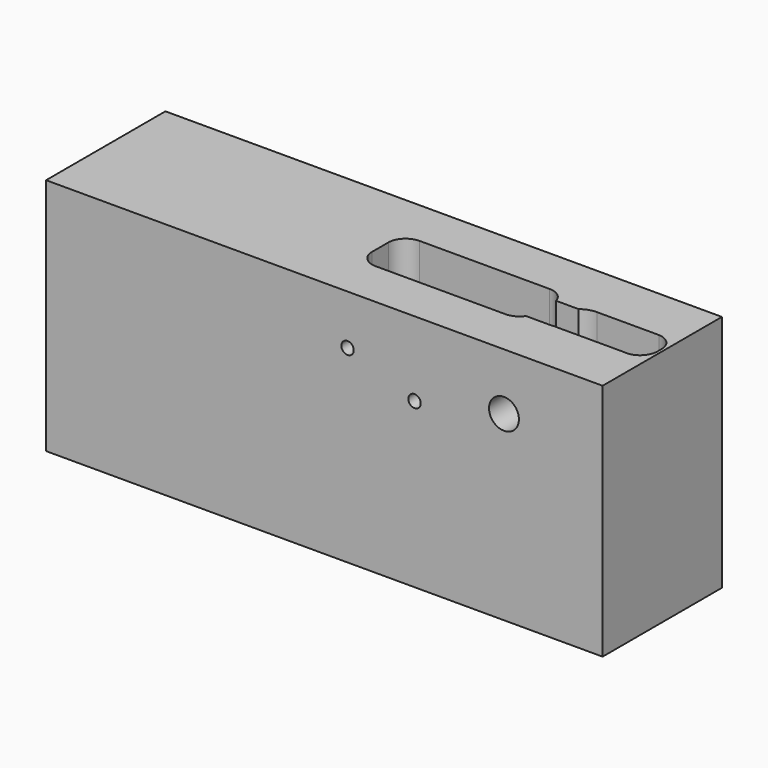
from build123d import *

# Parameters (mm, degrees)
F0_W      = 177.8
F0_H      = 47.6504
F1_DEPTH  = 76.2
F2_R      = 4.7752
F2_R_2    = 1.9812
F3_DEPTH  = 44.45
F5_DEPTH  = 16.002
F7_DEPTH  = 33.528
F9_DEPTH  = 31.7246
F11_DEPTH = 31.7246


# Not quite as in the source:
# - a feature names something its author has since deleted; it is built from what else it names


with BuildPart() as f1:
    # F0 (on Top) → F1 (new body)
    with BuildSketch(Plane.XY):
        with Locations((84.1375, 19.0627)):
            Rectangle(F0_W, F0_H)
    extrude(amount=-F1_DEPTH)

    # F2 (on face) → F3 (cut)
    with BuildSketch(Plane.XZ.offset(4.7625)):
        with Locations((141.5288, -18.1356)):
            Circle(F2_R)
        with Locations((112.9538, -23.8506)):
            Circle(F2_R_2)
        with Locations((91.5416, -15.875)):
            Circle(F2_R_2)
    extrude(amount=-F3_DEPTH, mode=Mode.SUBTRACT)

    # F4 (on face) → F5 (cut)
    with BuildSketch(Plane.XY):
        with BuildLine():
            Line((172.1358, 18.2664336953), (172.1358, 19.8998040895))
            ThreePointArc((172.1358, 19.8998040895), (170.6147547927, 23.7117700549), (166.887268424, 25.4294744577))
            Line((166.887268424, 25.4294744577), (147.1168, 25.4294744577))
            ThreePointArc((147.1168, 25.4294744577), (141.7286463274, 23.1976281303), (139.4968, 17.8094744577))
            Line((139.4968, 17.8094744577), (139.4968, 17.5517135975))
            ThreePointArc((139.4968, 17.5517135975), (140.8917039546, 14.1841175521), (144.2593, 12.7892135975))
            Line((144.2593, 12.7892135975), (165.7858, 12.7892135975))
            ThreePointArc((165.7858, 12.7892135975), (170.2152246474, 14.0735098945), (172.1358, 18.2664336953))
        make_face()
    extrude(amount=-F5_DEPTH, mode=Mode.SUBTRACT)

    # F6 (on face) → F7 (cut)
    with BuildSketch(Plane.XY):
        with BuildLine():
            Line((113.0554, 23.03145), (103.7082, 23.03145))
            ThreePointArc((103.7082, 23.03145), (100.9063600902, 21.8708899098), (99.7458, 19.06905))
            ThreePointArc((99.7458, 19.06905), (100.9063600902, 16.2672100902), (103.7082, 15.10665))
            Line((103.7082, 15.10665), (113.0554, 15.10665))
            ThreePointArc((113.0554, 15.10665), (115.8572399098, 16.2672100902), (117.0178, 19.06905))
            ThreePointArc((117.0178, 19.06905), (115.8572399098, 21.8708899098), (113.0554, 23.03145))
        make_face()
    extrude(amount=-F7_DEPTH, mode=Mode.SUBTRACT)

    # F8 (on face) → F9 (cut)
    with BuildSketch(Plane.XY):
        with BuildLine():
            Line((129.9972, 27.8257), (88.4682, 27.8257))
            ThreePointArc((88.4682, 27.8257), (84.5528083312, 26.2038916688), (82.931, 22.2885))
            Line((82.931, 22.2885), (82.931, 15.8369))
            ThreePointArc((82.931, 15.8369), (84.5528083312, 11.9215083312), (88.4682, 10.2997))
            Line((88.4682, 10.2997), (129.9972, 10.2997))
            ThreePointArc((129.9972, 10.2997), (133.9125916688, 11.9215083312), (135.5344, 15.8369))
            Line((135.5344, 15.8369), (135.5344, 22.2885))
            ThreePointArc((135.5344, 22.2885), (133.9125916688, 26.2038916688), (129.9972, 27.8257))
        make_face()
    extrude(amount=-F9_DEPTH, mode=Mode.SUBTRACT)

    # F10 (on face) → F11 (cut)
    with BuildSketch(Plane.XY):
        with BuildLine():
            Line((142.4686, 23.8379), (134.5240552125, 23.8379))
            ThreePointArc((134.5240552125, 23.8379), (132.2789911822, 22.9079640303), (131.3490552125, 20.6629))
            Line((131.3490552125, 20.6629), (131.3490552125, 15.8877))
            ThreePointArc((131.3490552125, 15.8877), (132.2789911822, 13.6426359697), (134.5240552125, 12.7127))
            Line((134.5240552125, 12.7127), (142.4686, 12.7127))
            ThreePointArc((142.4686, 12.7127), (146.3839916688, 14.3345083312), (148.0058, 18.2499))
            Line((148.0058, 18.2499), (148.0058, 18.3007))
            ThreePointArc((148.0058, 18.3007), (146.3839916688, 22.2160916688), (142.4686, 23.8379))
        make_face()
    extrude(amount=-F11_DEPTH, mode=Mode.SUBTRACT)


solid = f1.part
